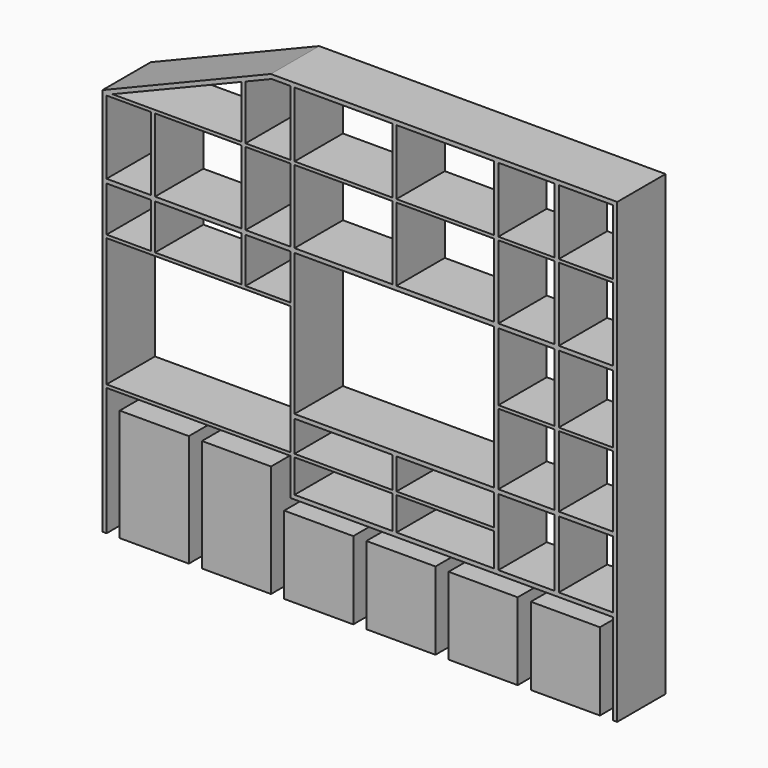
from build123d import *

# Parameters (mm, degrees)
F1_DEPTH = 350
F0_W     = 400
F0_H     = 450
F0_H_2   = 447.8067984339


# Not quite as in the source:
# - a feature names something its author has since deleted; it is built from what else it names


with BuildPart() as f1:
    # F0 (on Front) → F1 (new body)
    with BuildSketch(Plane.XZ):
        Polygon((0, 2249), (0, 0), (24, 0), (24, 502), (24, 741), (17, 741), (17, 759), (24, 759), (24, 1504.2), (17, 1504.2), (17, 1522.2), (24, 1522.2), (24, 1783), (17, 1783), (17, 1807), (24, 1807), (24, 2231), (17, 2231), (17, 2249), align=None)
        Polygon((0, 2251), (0, 2249), (17, 2249), (58.4801681387, 2249), (804.639455329, 2554.3513390656), (804.639455329, 2565.1562908123), (828.639455329, 2574.9778292739), (828.639455329, 2564.1728775272), (979.7207696423, 2626), (1088, 2626), (1088, 2636), (1112, 2636), (1112, 2626), (1678, 2626), (1678, 2636), (1702, 2636), (1702, 2626), (2268, 2626), (2268, 2636), (2291.9720954895, 2636), (2291.9720954895, 2626), (2618, 2626), (2618, 2636), (2642, 2636), (2642, 2626), (2956, 2626), (2980, 2650), (975, 2650), align=None)
        Polygon((58.4801681387, 2249), (17, 2249), (17, 2231), (24, 2231), (280.5054049087, 2231), (280.5054049087, 2236.0000610352), (304.5054049087, 2236.0000610352), (304.5054049087, 2231), (804.639455329, 2231), (811.639455329, 2231), (811.639455329, 2249), (804.639455329, 2249), (298.6695170403, 2249), align=None)
        Polygon((17, 741), (24, 741), (1088, 741), (1095, 741), (1095, 759), (1088, 759), (24, 759), (17, 759), align=None)
        Polygon((2980, 0), (2980, 2650), (2956, 2626), (2956, 2249), (2963, 2249), (2963, 2231), (2956, 2231), (2956, 1807), (2963, 1807), (2963, 1783), (2956, 1783), (2956, 1390.5), (2963, 1390.5), (2963, 1372.5), (2956, 1372.5), (2956, 962), (2963, 962), (2963, 938), (2956, 938), (2956, 550), (2963, 550), (2963, 526), (2956, 526), (2956, 502), (2956, 0), align=None)
        Polygon((804.639455329, 2565.1562908123), (804.639455329, 2554.3513390656), (804.639455329, 2249), (811.639455329, 2249), (811.639455329, 2231), (804.639455329, 2231), (804.639455329, 1807), (811.639455329, 1807), (811.639455329, 1783), (804.639455329, 1783), (804.639455329, 1522.2), (804.639455329, 1515.2), (828.639455329, 1515.2), (828.639455329, 1522.2), (828.639455329, 1783), (822.0379948616, 1783), (822.0379948616, 1807), (828.639455329, 1807), (828.639455329, 2231), (822.0379948616, 2231), (822.0379948616, 2249), (828.639455329, 2249), (828.639455329, 2564.1728775272), (828.639455329, 2574.9778292739), align=None)
        Polygon((1095, 741), (1088, 741), (1088, 526), (1112, 550), (1112, 741), (1105, 741), (1105, 759), (1112, 759), (1112, 938), (1105, 938), (1105, 962), (1112, 962), (1112, 1222.6), (1112, 1783), (1105, 1783), (1105, 1807), (1112, 1807), (1112, 2231), (1105, 2231), (1105, 2249), (1112, 2249), (1112, 2626), (1112, 2636), (1088, 2636), (1088, 2626), (1088, 2249), (1095, 2249), (1095, 2231), (1088, 2231), (1088, 1807), (1095, 1807), (1095, 1783), (1088, 1783), (1088, 1522.2), (1095, 1522.2), (1095, 1504.2), (1088, 1504.2), (1088, 1222.6), (1088, 938), (1088, 759), (1095, 759), align=None)
        Polygon((280.5054049087, 2236.0000610352), (280.5054049087, 2231), (280.5054049087, 1807), (287.3089313507, 1807), (287.3089313507, 1783), (280.5054049087, 1783), (280.5054049087, 1522.2), (280.5054049087, 1515.2), (304.5054049087, 1515.2), (304.5054049087, 1522.2), (304.5054049087, 1783), (298.6695170403, 1783), (298.6695170403, 1807), (304.5054049087, 1807), (304.5054049087, 2231), (304.5054049087, 2236.0000610352), align=None)
        Polygon((280.5054049087, 1807), (24, 1807), (17, 1807), (17, 1783), (24, 1783), (280.5054049087, 1783), (287.3089313507, 1783), (287.3089313507, 1807), align=None)
        Polygon((1112, 550), (1088, 526), (2956, 526), (2963, 526), (2963, 550), (2956, 550), (2642, 550), (2642, 540), (2618, 540), (2618, 550), (2292, 550), (2292, 540), (2268, 540), (2268, 550), (1702, 550), (1702, 540), (1678, 540), (1678, 550), align=None)
        Polygon((2642, 2249), (2642, 2626), (2642, 2636), (2618, 2636), (2618, 2626), (2618, 2249), (2625, 2249), (2625, 2231), (2618, 2231), (2618, 1807), (2625, 1807), (2625, 1783), (2618, 1783), (2618, 1390.5), (2625, 1390.5), (2625, 1372.5), (2618, 1372.5), (2618, 962), (2625, 962), (2625, 938), (2618, 938), (2618, 550), (2618, 540), (2642, 540), (2642, 550), (2642, 938), (2635, 938), (2635, 962), (2642, 962), (2642, 1372.5), (2635, 1372.5), (2635, 1390.5), (2642, 1390.5), (2642, 1783), (2635, 1783), (2635, 1807), (2642, 1807), (2642, 2231), (2635, 2231), (2635, 2249), align=None)
        Polygon((2963, 2249), (2956, 2249), (2642, 2249), (2635, 2249), (2635, 2231), (2642, 2231), (2956, 2231), (2963, 2231), align=None)
        Polygon((1678, 741), (1678, 550), (1678, 540), (1702, 540), (1702, 550), (1702, 741), (1695, 741), (1695, 759), (1702, 759), (1702, 938), (1702, 945), (1678, 945), (1678, 938), (1678, 759), (1685, 759), (1685, 741), align=None)
        Polygon((1105, 741), (1112, 741), (1678, 741), (1685, 741), (1685, 759), (1678, 759), (1112, 759), (1105, 759), align=None)
        Polygon((17, 1504.2), (24, 1504.2), (1088, 1504.2), (1095, 1504.2), (1095, 1522.2), (1088, 1522.2), (828.639455329, 1522.2), (828.639455329, 1515.2), (804.639455329, 1515.2), (804.639455329, 1522.2), (304.5054049087, 1522.2), (304.5054049087, 1515.2), (280.5054049087, 1515.2), (280.5054049087, 1522.2), (24, 1522.2), (17, 1522.2), align=None)
        Polygon((1088, 2249), (828.639455329, 2249), (822.0379948616, 2249), (822.0379948616, 2231), (828.639455329, 2231), (1088, 2231), (1095, 2231), (1095, 2249), align=None)
        Polygon((811.639455329, 1807), (804.639455329, 1807), (304.5054049087, 1807), (298.6695170403, 1807), (298.6695170403, 1783), (304.5054049087, 1783), (804.639455329, 1783), (811.639455329, 1783), align=None)
        Polygon((2291.9720954895, 2249), (2291.9720954895, 2626), (2291.9720954895, 2636), (2268, 2636), (2268, 2626), (2268, 2249), (2275, 2249), (2275, 2231), (2268, 2231), (2268, 1807), (2275, 1807), (2275, 1783), (2268, 1783), (2268, 962), (2275, 962), (2275, 938), (2268, 938), (2268, 759), (2275, 759), (2275, 741), (2268, 741), (2268, 550), (2268, 540), (2292, 540), (2292, 550), (2292, 938), (2284.9720954895, 938), (2284.9720954895, 962), (2292, 962), (2292, 1372.5), (2284.9720954895, 1372.5), (2284.9720954895, 1390.5), (2292, 1390.5), (2292, 1783), (2284.9720954895, 1783), (2284.9720954895, 1807), (2291.9720954895, 1807), (2291.9720954895, 2231), (2284.9720954895, 2231), (2284.9720954895, 2249), align=None)
        Polygon((2625, 2249), (2618, 2249), (2291.9720954895, 2249), (2284.9720954895, 2249), (2284.9720954895, 2231), (2291.9720954895, 2231), (2618, 2231), (2625, 2231), align=None)
        Polygon((2963, 1807), (2956, 1807), (2642, 1807), (2635, 1807), (2635, 1783), (2642, 1783), (2818.1127872467, 1783), (2956, 1783), (2963, 1783), align=None)
        Polygon((2642, 938), (2956, 938), (2963, 938), (2963, 962), (2956, 962), (2818.1127872467, 962), (2642, 962), (2635, 962), (2635, 938), align=None)
        Polygon((1695, 741), (1702, 741), (2268, 741), (2275, 741), (2275, 759), (2268, 759), (1702, 759), (1695, 759), align=None)
        Polygon((1105, 938), (1112, 938), (1678, 938), (1678, 945), (1702, 945), (1702, 938), (2268, 938), (2275, 938), (2275, 962), (2268, 962), (1112, 962), (1105, 962), align=None)
        Polygon((1088, 1807), (828.639455329, 1807), (822.0379948616, 1807), (822.0379948616, 1783), (828.639455329, 1783), (1088, 1783), (1095, 1783), (1095, 1807), align=None)
        Polygon((1678, 2636), (1678, 2626), (1678, 2249), (1685, 2249), (1685, 2231), (1678, 2231), (1678, 1807), (1678, 1800), (1702, 1800), (1702, 1807), (1702, 2231), (1695, 2231), (1695, 2249), (1702, 2249), (1702, 2626), (1702, 2636), align=None)
        Polygon((1678, 2249), (1112, 2249), (1105, 2249), (1105, 2231), (1112, 2231), (1678, 2231), (1685, 2231), (1685, 2249), align=None)
        Polygon((2275, 2249), (2268, 2249), (1702, 2249), (1695, 2249), (1695, 2231), (1702, 2231), (2268, 2231), (2275, 2231), align=None)
        Polygon((2625, 1807), (2618, 1807), (2291.9720954895, 1807), (2284.9720954895, 1807), (2284.9720954895, 1783), (2292, 1783), (2618, 1783), (2625, 1783), align=None)
        Polygon((2963, 1390.5), (2956, 1390.5), (2642, 1390.5), (2635, 1390.5), (2635, 1372.5), (2642, 1372.5), (2956, 1372.5), (2963, 1372.5), align=None)
        Polygon((2292, 938), (2618, 938), (2625, 938), (2625, 962), (2618, 962), (2292, 962), (2284.9720954895, 962), (2284.9720954895, 938), align=None)
        Polygon((1112, 1783), (2268, 1783), (2275, 1783), (2275, 1807), (2268, 1807), (1702, 1807), (1702, 1800), (1678, 1800), (1678, 1807), (1112, 1807), (1105, 1807), (1105, 1783), align=None)
        Polygon((2625, 1390.5), (2618, 1390.5), (2292, 1390.5), (2284.9720954895, 1390.5), (2284.9720954895, 1372.5), (2292, 1372.5), (2618, 1372.5), (2625, 1372.5), align=None)
    extrude(amount=F1_DEPTH)


with BuildPart() as f1b:
    # F0 (on Front) → F1, piece 2 (new body)
    with BuildSketch(Plane.XZ):
        Polygon((100, 450), (100, 0), (500, 0), (500, 450), (500, 650), (100, 650), align=None)
    extrude(amount=F1_DEPTH)


with BuildPart() as f1c:
    # F0 (on Front) → F1, piece 3 (new body)
    with BuildSketch(Plane.XZ):
        Polygon((576, 450), (576, 0), (976, 0), (976, 450), (976, 650), (576, 650), align=None)
    extrude(amount=F1_DEPTH)


with BuildPart() as f1d:
    # F0 (on Front) → F1, piece 4 (new body)
    with BuildSketch(Plane.XZ):
        with Locations((1252, 225)):
            Rectangle(F0_W, F0_H)
    extrude(amount=F1_DEPTH)


with BuildPart() as f1e:
    # F0 (on Front) → F1, piece 5 (new body)
    with BuildSketch(Plane.XZ):
        Polygon((2850, 0), (2880, 0), (2880, 450), (2480, 450), (2480, 0), align=None)
    extrude(amount=F1_DEPTH)


with BuildPart() as f1f:
    # F0 (on Front) → F1, piece 6 (new body)
    with BuildSketch(Plane.XZ):
        with Locations((1728, 225)):
            Rectangle(F0_W, F0_H)
    extrude(amount=F1_DEPTH)


with BuildPart() as f1g:
    # F0 (on Front) → F1, piece 7 (new body)
    with BuildSketch(Plane.XZ):
        with Locations((2204, 223.9033992169)):
            Rectangle(F0_W, F0_H_2)
    extrude(amount=F1_DEPTH)


solid = Compound([f1.part, f1b.part, f1c.part, f1d.part, f1e.part, f1f.part, f1g.part])
